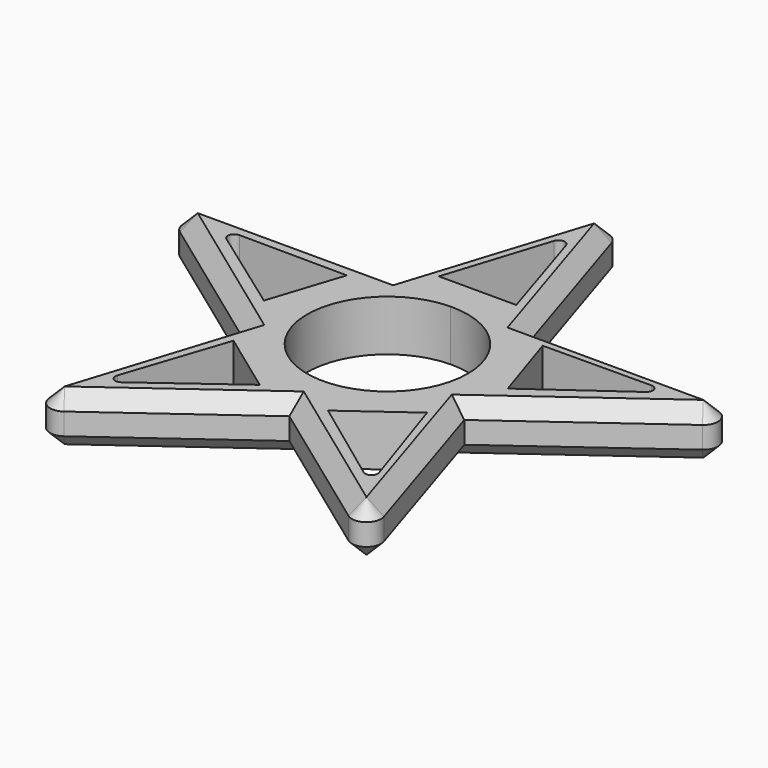
from build123d import *

# Parameters (mm, degrees)
F1_DEPTH = 7
F2_R     = 2
F3_R     = 0.8678369572
F4_SIZE  = 1.99999
F5_SIZE  = 1.99999


# Not quite as in the source:
# - a fillet or chamfer is up to 0.001 mm smaller than in the source, because OpenCascade refuses the exact size


with BuildPart() as f1:
    # F0 (on Top) → F1 (new body)
    with BuildSketch(Plane.XY):
        Polygon((9.1365975469, 13.0565894232), (-0.1652448664, 13.0565894232), (-9.5275098884, 13.0565894232), (-15.4519321666, -5.5724489729), (-0.1296436349, -16.7047432175), (15.0836615604, -5.6335964123), align=None)
        with BuildLine():
            ThreePointArc((-0.1630055447, 11.0487976356), (7.7556846484, 7.87095011), (11.05, 0))
            ThreePointArc((11.05, 0), (-7.7556846484, -7.87095011), (-0.1630055447, 11.0487976356))
        make_face(mode=Mode.SUBTRACT)
        Polygon((-9.5275098884, 13.0565894232), (-0.1652448664, 13.0565894232), (-0.1682447051, 15.7462661459), (-5.5240840498, 15.7462661459), (-0.1869622706, 32.5285686018), (-0.1979640721, 42.3928620705), align=None)
        Polygon((-0.1682447051, 15.7462661459), (-0.1652448664, 13.0565894232), (9.1365975469, 13.0565894232), (-0.1979640721, 42.3928620705), (-0.1869622706, 32.5285686018), (5.1325563495, 15.7462661459), align=None)
        Polygon((-15.4519321666, -5.5724489729), (-9.5275098884, 13.0565894232), (-41.0926038108, 13.0565894232), align=None)
        Polygon((-16.6826248751, -0.3878522951), (-30.9942816534, 9.8740688149), (-13.3895418888, 9.7472149984), align=None, mode=Mode.SUBTRACT)
        Polygon((40.7665927214, 13.0565894232), (9.1365975469, 13.0565894232), (15.0836615604, -5.6335964123), align=None)
        Polygon((13.2685531756, 10.1195799691), (30.8787326155, 10.2296921864), (16.561636162, -0.0154873244), align=None, mode=Mode.SUBTRACT)
        Polygon((-0.1296436349, -16.7047432175), (-15.4519321666, -5.5724489729), (-24.67217675, -34.5650295656), align=None)
        Polygon((-4.7863451446, -15.9859720469), (-18.9685572481, -26.4260584669), (-13.4077483305, -9.7221559812), align=None, mode=Mode.SUBTRACT)
        Polygon((24.2402355164, -34.4104968233), (15.0836615604, -5.6335964123), (-0.1296436349, -16.7047432175), align=None)
        Polygon((13.3053196858, -9.8071458261), (18.8518873485, -26.5213951891), (4.6839164999, -16.0709618918), align=None, mode=Mode.SUBTRACT)
    extrude(amount=F1_DEPTH)

    # F2
    f2_edges = [f1.edges().sort_by_distance(p)[0] for p in [
        (-0.197964, 42.392862, 3.5),
        (40.766593, 13.056589, 3.5),
        (24.240236, -34.410497, 3.5),
        (-24.672177, -34.56503, 3.5),
        (-41.092604, 13.056589, 3.5),
    ]]
    fillet(f2_edges, radius=F2_R)

    # F3
    f3_edges = [f1.edges().sort_by_distance(p)[0] for p in [
        (-18.968557, -26.426058, 3.5),
        (-30.994282, 9.874069, 3.5),
        (18.851887, -26.521395, 3.5),
        (30.878733, 10.229692, 3.5),
        (-0.186962, 32.528569, 3.5),
    ]]
    fillet(f3_edges, radius=F3_R)

    # F4 (size 2 in the source; OpenCascade refuses exactly that, so slightly less here)
    f4_edges = [f1.edges().sort_by_distance(p)[0] for p in [
        (-22.232373, 13.056589, 7),
        (-5.815451, 24.728966, 7),
        (-0.197607, 37.795214, 7),
        (5.422496, 24.729114, 7),
        (21.877967, 13.056589, 7),
        (36.521209, 11.675361, 7),
        (25.439911, 1.902936, 7),
        (18.738348, -17.119392, 7),
        (21.65782, -30.833222, 7),
        (9.590987, -23.767195, 7),
        (-9.935411, -23.840674, 7),
        (-19.137937, -17.162901, 7),
        (-25.78237, 1.933053, 7),
        (-36.83935, 11.674623, 7),
    ]]
    chamfer(f4_edges, length=F4_SIZE)

    # F5 (size 2 in the source; OpenCascade refuses exactly that, so slightly less here)
    f5_edges = [f1.edges().sort_by_distance(p)[0] for p in [
        (21.877967, 13.056589, 0),
        (5.422496, 24.729114, 0),
        (-5.815451, 24.728966, 0),
        (-22.232373, 13.056589, 0),
        (-25.78237, 1.933053, 0),
        (-19.137937, -17.162901, 0),
        (-9.935411, -23.840674, 0),
        (9.590987, -23.767195, 0),
        (25.439911, 1.902936, 0),
        (18.738348, -17.119392, 0),
        (-36.83935, 11.674623, 0),
        (-0.197607, 37.795214, 0),
        (36.521209, 11.675361, 0),
        (21.65782, -30.833222, 0),
        (-22.08788, -30.981637, 0),
    ]]
    chamfer(f5_edges, length=F5_SIZE)


solid = f1.part
